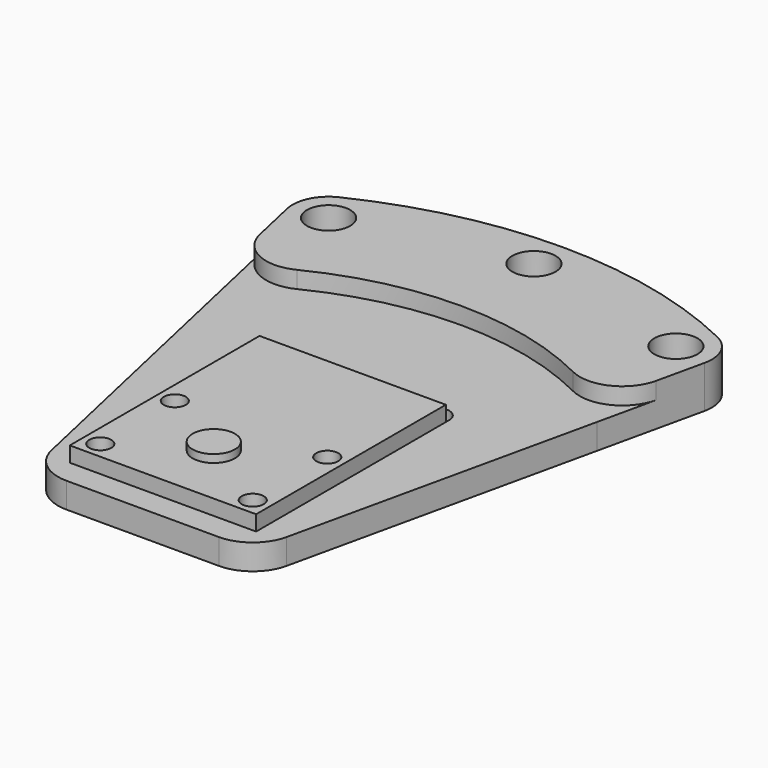
from build123d import *

# Parameters (mm, degrees)
F0_W     = 22
F0_H     = 28
F0_R     = 1.3
F0_R_2   = 2.5
F1_DEPTH = 1.8
F2_R     = 2.5
F3_DEPTH = 2.73
F4_R     = 2.55
F4_W     = 22
F4_H     = 21
F4_R_2   = 1.3
F5_DEPTH = 3
F6_DEPTH = 2
F7_R     = 5
F8_R     = 1.5


with BuildPart() as f1:
    # F0 (on Top) → F1 (new body)
    with BuildSketch(Plane.XY):
        with Locations((0, 6.5)):
            Rectangle(F0_W, F0_H)
        with Locations((-9, -5.5)):
            Circle(F0_R, mode=Mode.SUBTRACT)
        with Locations((-9, 5.5)):
            Circle(F0_R, mode=Mode.SUBTRACT)
        with Locations((9, -5.5)):
            Circle(F0_R, mode=Mode.SUBTRACT)
        Circle(F0_R_2, mode=Mode.SUBTRACT)
        with Locations((9, 5.5)):
            Circle(F0_R, mode=Mode.SUBTRACT)
    extrude(amount=F1_DEPTH)

    # F2 (on face) → F3 (join)
    with BuildSketch(Plane(origin=(0, 0, 0), x_dir=(1, 0, 0), z_dir=(0, 0, -1))):
        Circle(F2_R)
    extrude(amount=-F3_DEPTH)


with BuildPart() as f5:
    # F4 (on face) → F5 (new body)
    with BuildSketch(Plane(origin=(0, 0, 0), x_dir=(1, 0, 0), z_dir=(0, 0, -1))):
        with BuildLine():
            Line((9, 10.5), (-9, 10.5))
            ThreePointArc((-9, 10.5), (-12.1267541127, 9.4017186878), (-13.8798859815, 6.5893634874))
            Line((-13.8798859815, 6.5893634874), (-21.8737337821, -29.2196812171))
            ThreePointArc((-21.8737337821, -29.2196812171), (0, -36.5), (21.8737337821, -29.2196812171))
            Line((21.8737337821, -29.2196812171), (13.8798859815, 6.5893634874))
            ThreePointArc((13.8798859815, 6.5893634874), (12.1267541127, 9.4017186878), (9, 10.5))
        make_face()
        Polygon((-11, -20.5), (-11, -13.5), (-11, 7.5), (11, 7.5), (11, -13.5), (11, -20.5), (11, -22.5), (-11, -22.5), align=None, mode=Mode.SUBTRACT)
        with BuildLine():
            ThreePointArc((21.8737337821, -29.2196812171), (0, -36.5), (-21.8737337821, -29.2196812171))
            Line((-21.8737337821, -29.2196812171), (-24.6479511299, -41.6469972609))
            ThreePointArc((-24.6479511299, -41.6469972609), (-24.324916161, -44.4247666907), (-22.3451494117, -46.3998307946))
            ThreePointArc((-22.3451494117, -46.3998307946), (0, -51.5), (22.3451494117, -46.3998307946))
            ThreePointArc((22.3451494117, -46.3998307946), (24.324916161, -44.4247666907), (24.6479511299, -41.6469972609))
            Line((24.6479511299, -41.6469972609), (21.8737337821, -29.2196812171))
        make_face()
        with Locations((-20.502, -42.5725204798)):
            Circle(F4_R, mode=Mode.SUBTRACT)
        with Locations((0, -47.252)):
            Circle(F4_R, mode=Mode.SUBTRACT)
        with Locations((20.502, -42.5725204798)):
            Circle(F4_R, mode=Mode.SUBTRACT)
        with Locations((0, -3)):
            Rectangle(F4_W, F4_H)
        with Locations((-9, -5.5)):
            Circle(F4_R_2, mode=Mode.SUBTRACT)
        with Locations((-9, 5.5)):
            Circle(F4_R_2, mode=Mode.SUBTRACT)
        with Locations((9, -5.5)):
            Circle(F4_R_2, mode=Mode.SUBTRACT)
        with Locations((9, 5.5)):
            Circle(F4_R_2, mode=Mode.SUBTRACT)
    extrude(amount=F5_DEPTH)

    # F4 (on face) → F6 (join)
    with BuildSketch(Plane(origin=(0, 0, 0), x_dir=(1, 0, 0), z_dir=(0, 0, -1))):
        with BuildLine():
            ThreePointArc((21.8737337821, -29.2196812171), (0, -36.5), (-21.8737337821, -29.2196812171))
            Line((-21.8737337821, -29.2196812171), (-24.6479511299, -41.6469972609))
            ThreePointArc((-24.6479511299, -41.6469972609), (-24.324916161, -44.4247666907), (-22.3451494117, -46.3998307946))
            ThreePointArc((-22.3451494117, -46.3998307946), (0, -51.5), (22.3451494117, -46.3998307946))
            ThreePointArc((22.3451494117, -46.3998307946), (24.324916161, -44.4247666907), (24.6479511299, -41.6469972609))
            Line((24.6479511299, -41.6469972609), (21.8737337821, -29.2196812171))
        make_face()
        with Locations((-20.502, -42.5725204798)):
            Circle(F4_R, mode=Mode.SUBTRACT)
        with Locations((0, -47.252)):
            Circle(F4_R, mode=Mode.SUBTRACT)
        with Locations((20.502, -42.5725204798)):
            Circle(F4_R, mode=Mode.SUBTRACT)
    extrude(amount=-F6_DEPTH)

    # F7
    f7_edges = [f5.edges().sort_by_distance(p)[0] for p in [
        (21.873734, 29.219681, 1),
        (-21.873734, 29.219681, 1),
    ]]
    fillet(f7_edges, radius=F7_R)

    # F8
    f8_edges = [f5.edges().sort_by_distance(p)[0] for p in [
        (11, 22.5, -1.5),
        (11, 13.5, -1.5),
        (-11, 22.5, -1.5),
        (-11, 13.5, -1.5),
    ]]
    fillet(f8_edges, radius=F8_R)


solid = Compound([f1.part, f5.part])
